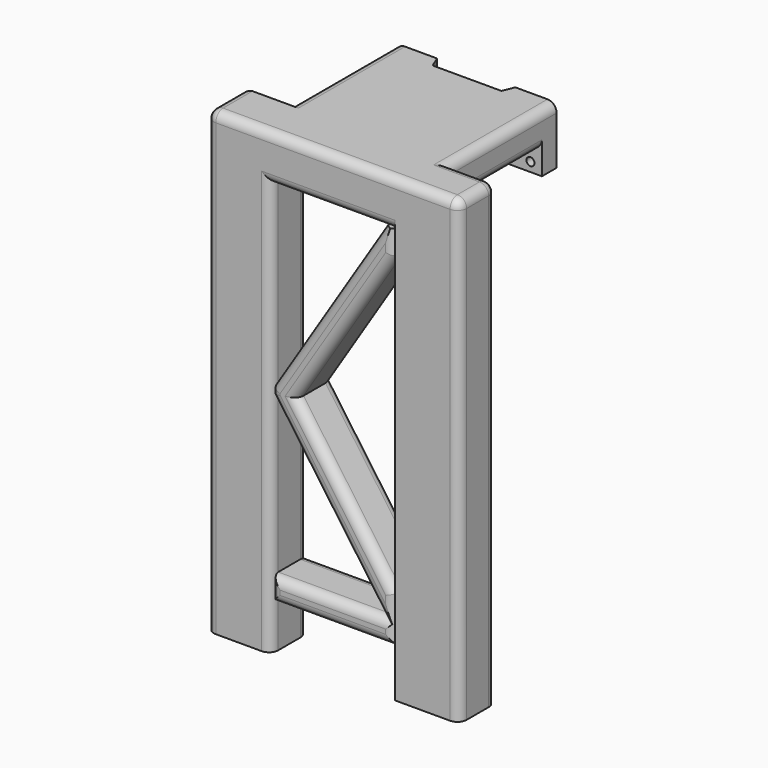
from build123d import *

# Parameters (mm, degrees)
F1_DEPTH         = 25
F2_R             = 1.75
F3_DEPTH         = 25
F4_W             = 70
F4_H             = 15
F5_DEPTH         = 50
F7_DEPTH         = 20
F7_DEPTH_BACK    = 90
F8_W             = 54
F8_H             = 180
F9_DEPTH         = 25
F12_DEPTH        = 20
F13_DEPTH        = 25
F14_T1_DEPTH     = 190
F14_T3_DEPTH     = 220
F14_T5_DEPTH     = 206
F14_T7_DEPTH     = 102
F14_T9_DEPTH     = 12
F14_T11_DEPTH    = 16
F14_T13_DEPTH    = 68
F14_T15_DEPTH    = 50
F14_T17_DEPTH    = 54
F14_T19_DEPTH    = 26
F14_S23_W        = 4
F14_S23_H        = 4
F14_T24_DEPTH    = 4
F14_S29_W        = 4
F14_S29_H        = 4
F14_T30_DEPTH    = 4
F14_S35_W        = 4
F14_S35_H        = 4
F14_T36_DEPTH    = 4
F14_T43_DEPTH    = 200
F14_T48_DEPTH    = 64
F14_T55_DEPTH    = 64
F14_T59_DEPTH    = 200
F14_T67_DEPTH    = 200
F14_T71_DEPTH    = 64
F14_T78_DEPTH    = 26
F14_T82_DEPTH    = 78
F14_2_T1_DEPTH   = 111.7221358849
F14_2_T3_DEPTH   = 30
F14_2_T5_DEPTH   = 74
F14_2_T7_DEPTH   = 40.2556151979
F14_2_T9_DEPTH   = 30.8068882586
F14_2_T11_DEPTH  = 23.071224869
F14_2_T16_DEPTH  = 100.4908539398
F14_2_T21_DEPTH  = 100.4908539398
F14_2_T26_DEPTH  = 94.5466591948
F14_2_T31_DEPTH  = 94.5466591948
F14_2_T36_DEPTH  = 104.9485186174
F14_2_T41_DEPTH  = 104.9485186174
F14_2_T46_DEPTH  = 69
F14_2_T51_DEPTH  = 69
F14_2_T57_DEPTH  = 94.5466591948
F14_2_T62_DEPTH  = 100.4908539398
F14_2_T70_DEPTH  = 100.4908539398
F14_2_T75_DEPTH  = 94.5466591948
F14_2_T83_DEPTH  = 59
F14_2_T88_DEPTH  = 104.9485186174
F14_2_T96_DEPTH  = 59
F14_2_T101_DEPTH = 104.9485186174


# Not quite as in the source:
# - a fillet or chamfer that OpenCascade refuses, or shapes differently, is made with other operations: its cross-section is extruded or revolved along the edge and cut away or added


with BuildPart() as f1:
    # F0 (on Top) → F1 (new body)
    with BuildSketch(Plane.XY):
        Polygon((-30.8332282406, 24.8506308587), (-48.8332282406, 24.8506308587), (-48.8332282406, 16.8506308587), (21.1667717594, 16.8506308587), (21.1667717594, 24.8506308587), (3.1667717594, 24.8506308587), (1.1667717594, 19.8506308587), (-28.8332282406, 19.8506308587), align=None)
    extrude(amount=F1_DEPTH)

    # F2 (on face) → F3 (cut)
    with BuildSketch(Plane(origin=(0, 24.8506308587, 0), x_dir=(-1, 0, 0), z_dir=(0, 1, 0))):
        with Locations((-16.1667717594, 4)):
            Circle(F2_R)
        with Locations((43.8332282406, 4)):
            Circle(F2_R)
    extrude(amount=-F3_DEPTH, mode=Mode.SUBTRACT)

    # F4 (on face) → F5 (join)
    with BuildSketch(Plane.XZ.offset(-16.8506308587)):
        with Locations((-13.8332282406, 17.5)):
            Rectangle(F4_W, F4_H)
    extrude(amount=F5_DEPTH)

    # F6 (on face) → F7 (join, two sides)
    with BuildSketch(Plane.YZ.offset(21.1667717594)) as f7_sk:
        Polygon((-33.1493691413, 10), (-33.1493691413, 25), (-53.1493691413, 25), (-53.1493691413, -175), (-33.1493691413, -175), align=None)
    extrude(amount=F7_DEPTH)
    extrude(f7_sk.sketch, amount=-F7_DEPTH_BACK)

    # F8 (on face) → F9 (cut)
    with BuildSketch(Plane(origin=(0, -33.1493691413, 0), x_dir=(-1, 0, 0), z_dir=(0, 1, 0))):
        with Locations((13.8332282406, -85)):
            Rectangle(F8_W, F8_H)
    extrude(amount=-F9_DEPTH, mode=Mode.SUBTRACT)

    # F10 (on face) → F13 (cut)
    with BuildSketch(Plane(origin=(0, 0, -175), x_dir=(1, 0, 0), z_dir=(0, 0, -1))):
        with BuildLine():
            Line((-62.8332282406, 37.1493691413), (-46.8332282406, 37.1493691413))
            ThreePointArc((-46.8332282406, 37.1493691413), (-45.4190146782, 37.7351555789), (-44.8332282406, 39.1493691413))
            Line((-44.8332282406, 39.1493691413), (-44.8332282406, 47.1493691413))
            ThreePointArc((-44.8332282406, 47.1493691413), (-45.4190146782, 48.5635827036), (-46.8332282406, 49.1493691413))
            Line((-46.8332282406, 49.1493691413), (-62.8332282406, 49.1493691413))
            ThreePointArc((-62.8332282406, 49.1493691413), (-64.247441803, 48.5635827036), (-64.8332282406, 47.1493691413))
            Line((-64.8332282406, 47.1493691413), (-64.8332282406, 39.1493691413))
            ThreePointArc((-64.8332282406, 39.1493691413), (-64.247441803, 37.7351555789), (-62.8332282406, 37.1493691413))
        make_face()
        with BuildLine():
            Line((19.1667717594, 37.1493691413), (35.1667717594, 37.1493691413))
            ThreePointArc((35.1667717594, 37.1493691413), (36.5809853218, 37.7351555789), (37.1667717594, 39.1493691413))
            Line((37.1667717594, 39.1493691413), (37.1667717594, 47.1493691413))
            ThreePointArc((37.1667717594, 47.1493691413), (36.5809853218, 48.5635827036), (35.1667717594, 49.1493691413))
            Line((35.1667717594, 49.1493691413), (19.1667717594, 49.1493691413))
            ThreePointArc((19.1667717594, 49.1493691413), (17.752558197, 48.5635827036), (17.1667717594, 47.1493691413))
            Line((17.1667717594, 47.1493691413), (17.1667717594, 39.1493691413))
            ThreePointArc((17.1667717594, 39.1493691413), (17.752558197, 37.7351555789), (19.1667717594, 37.1493691413))
        make_face()
    extrude(amount=-F13_DEPTH, mode=Mode.SUBTRACT)

    # F14: fillet of radius 4 on 17 edges, made by hand

    # F14_s2 → F14_t1 (cut)
    with BuildSketch(Plane.XY.offset(-185)):
        with BuildLine():
            ThreePointArc((13.1667717594, -37.1493691413), (14.3383446347, -34.3209420165), (17.1667717594, -33.1493691413))
            Line((17.1667717594, -33.1493691413), (13.1667717594, -33.1493691413))
            Line((13.1667717594, -33.1493691413), (13.1667717594, -37.1493691413))
        make_face()
        with BuildLine():
            ThreePointArc((-44.8332282406, -33.1493691413), (-42.0048011158, -34.3209420165), (-40.8332282406, -37.1493691413))
            Line((-40.8332282406, -37.1493691413), (-40.8332282406, -33.1493691413))
            Line((-40.8332282406, -33.1493691413), (-44.8332282406, -33.1493691413))
        make_face()
        with BuildLine():
            ThreePointArc((-44.8332282406, -53.1493691413), (-42.0048011158, -51.977796266), (-40.8332282406, -49.1493691413))
            Line((-40.8332282406, -49.1493691413), (-40.8332282406, -53.1493691413))
            Line((-40.8332282406, -53.1493691413), (-44.8332282406, -53.1493691413))
        make_face()
    extrude(amount=F14_T1_DEPTH, mode=Mode.SUBTRACT)

    # F14_s4 → F14_t3 (cut)
    with BuildSketch(Plane.XY.offset(-185)):
        with BuildLine():
            ThreePointArc((-64.8332282406, -33.1493691413), (-67.6616553653, -34.3209420165), (-68.8332282406, -37.1493691413))
            Line((-68.8332282406, -37.1493691413), (-68.8332282406, -33.1493691413))
            Line((-68.8332282406, -33.1493691413), (-64.8332282406, -33.1493691413))
        make_face()
    extrude(amount=F14_T3_DEPTH, mode=Mode.SUBTRACT)

    # F14_s6 → F14_t5 (cut)
    with BuildSketch(Plane.XY.offset(-185)):
        with BuildLine():
            ThreePointArc((41.1667717594, -37.1493691413), (39.9951988842, -34.3209420165), (37.1667717594, -33.1493691413))
            Line((37.1667717594, -33.1493691413), (41.1667717594, -33.1493691413))
            Line((41.1667717594, -33.1493691413), (41.1667717594, -37.1493691413))
        make_face()
        with BuildLine():
            ThreePointArc((37.1667717594, -53.1493691413), (39.9951988842, -51.977796266), (41.1667717594, -49.1493691413))
            Line((41.1667717594, -49.1493691413), (41.1667717594, -53.1493691413))
            Line((41.1667717594, -53.1493691413), (37.1667717594, -53.1493691413))
        make_face()
        with BuildLine():
            ThreePointArc((-64.8332282406, -53.1493691413), (-67.6616553653, -51.977796266), (-68.8332282406, -49.1493691413))
            Line((-68.8332282406, -49.1493691413), (-68.8332282406, -53.1493691413))
            Line((-68.8332282406, -53.1493691413), (-64.8332282406, -53.1493691413))
        make_face()
    extrude(amount=F14_T5_DEPTH, mode=Mode.SUBTRACT)

    # F14_s8 → F14_t7 (cut)
    with BuildSketch(Plane.YZ.offset(-64.8332282406)):
        with BuildLine():
            ThreePointArc((-53.1493691413, 21), (-51.977796266, 23.8284271247), (-49.1493691413, 25))
            Line((-49.1493691413, 25), (-53.1493691413, 25))
            Line((-53.1493691413, 25), (-53.1493691413, 21))
        make_face()
    extrude(amount=F14_T7_DEPTH, mode=Mode.SUBTRACT)

    # F14_s10 → F14_t9 (cut)
    with BuildSketch(Plane.XZ.offset(37.1493691413)):
        with BuildLine():
            ThreePointArc((41.1667717594, 21), (39.9951988842, 23.8284271247), (37.1667717594, 25))
            Line((37.1667717594, 25), (41.1667717594, 25))
            Line((41.1667717594, 25), (41.1667717594, 21))
        make_face()
    extrude(amount=F14_T9_DEPTH, mode=Mode.SUBTRACT)

    # F14_s12 → F14_t11 (cut)
    with BuildSketch(Plane.YZ.offset(21.1667717594)):
        with BuildLine():
            ThreePointArc((-33.1493691413, 21), (-34.3209420165, 23.8284271247), (-37.1493691413, 25))
            Line((-37.1493691413, 25), (-33.1493691413, 25))
            Line((-33.1493691413, 25), (-33.1493691413, 21))
        make_face()
    extrude(amount=F14_T11_DEPTH, mode=Mode.SUBTRACT)

    # F14_s14 → F14_t13 (cut)
    with BuildSketch(Plane.XZ.offset(-34.8506308587)):
        with BuildLine():
            ThreePointArc((17.1667717594, 25), (19.9951988842, 23.8284271247), (21.1667717594, 21))
            Line((21.1667717594, 21), (21.1667717594, 25))
            Line((21.1667717594, 25), (17.1667717594, 25))
        make_face()
        with BuildLine():
            ThreePointArc((-44.8332282406, 25), (-47.6616553653, 23.8284271247), (-48.8332282406, 21))
            Line((-48.8332282406, 21), (-48.8332282406, 25))
            Line((-48.8332282406, 25), (-44.8332282406, 25))
        make_face()
    extrude(amount=F14_T13_DEPTH, mode=Mode.SUBTRACT)

    # F14_s16 → F14_t15 (cut)
    with BuildSketch(Plane.XZ.offset(-16.8506308587)):
        with BuildLine():
            ThreePointArc((17.1667717594, 10), (19.9951988842, 11.1715728753), (21.1667717594, 14))
            Line((21.1667717594, 14), (21.1667717594, 10))
            Line((21.1667717594, 10), (17.1667717594, 10))
        make_face()
        with BuildLine():
            ThreePointArc((-48.8332282406, 14), (-47.6616553653, 11.1715728753), (-44.8332282406, 10))
            Line((-44.8332282406, 10), (-48.8332282406, 10))
            Line((-48.8332282406, 10), (-48.8332282406, 14))
        make_face()
    extrude(amount=F14_T15_DEPTH, mode=Mode.SUBTRACT)

    # F14_s18 → F14_t17 (cut)
    with BuildSketch(Plane.YZ.offset(-40.8332282406)):
        with BuildLine():
            ThreePointArc((-53.1493691413, 9), (-51.977796266, 6.1715728753), (-49.1493691413, 5))
            Line((-49.1493691413, 5), (-53.1493691413, 5))
            Line((-53.1493691413, 5), (-53.1493691413, 9))
        make_face()
        with BuildLine():
            ThreePointArc((-33.1493691413, 9), (-34.3209420165, 6.1715728753), (-37.1493691413, 5))
            Line((-37.1493691413, 5), (-33.1493691413, 5))
            Line((-33.1493691413, 5), (-33.1493691413, 9))
        make_face()
    extrude(amount=F14_T17_DEPTH, mode=Mode.SUBTRACT)

    # F14_s20 → F14_t19 (cut)
    with BuildSketch(Plane.XZ.offset(23.1493691413)):
        with BuildLine():
            ThreePointArc((-64.8332282406, 25), (-67.6616553653, 23.8284271247), (-68.8332282406, 21))
            Line((-68.8332282406, 21), (-68.8332282406, 25))
            Line((-68.8332282406, 25), (-64.8332282406, 25))
        make_face()
    extrude(amount=F14_T19_DEPTH, mode=Mode.SUBTRACT)


with BuildPart() as f12:
    # F11 (on face) → F12 (new body)
    with BuildSketch(Plane.XZ.offset(53.1493691413)):
        Polygon((-40.8332282406, -145), (-40.8332282406, -155), (13.1667717594, -155), (13.1667717594, -145), (13.1667717594, -134.7443848021), (-29.8332282406, -73.8493571142), (13.1667717594, -5.8068882586), (13.1667717594, 5), (8.1667717594, 5), (-40.8332282406, -72.5367668354), (-40.8332282406, -75.6079917045), (8.1667717594, -145), align=None)
    extrude(amount=-F12_DEPTH)

    # F14#2: fillet of radius 4 on 17 edges, made by hand

    # F14_2_s2 → F14_2_t1 (cut)
    with BuildSketch(Plane(origin=(9.9309720555, 0, 15.7146013207), x_dir=(0, 1, 0), z_dir=(-0.5342221867, 0, -0.8453441046))):
        with BuildLine():
            ThreePointArc((-33.1493691413, 8.2326214273), (-34.3209420165, 5.4041943026), (-37.1493691413, 4.2326214273))
            Line((-37.1493691413, 4.2326214273), (-33.1493691413, 4.2326214273))
            Line((-33.1493691413, 4.2326214273), (-33.1493691413, 8.2326214273))
        make_face()
        with BuildLine():
            ThreePointArc((-49.1493691413, 4.2326214273), (-51.977796266, 5.4041943026), (-53.1493691413, 8.2326214273))
            Line((-53.1493691413, 8.2326214273), (-53.1493691413, 4.2326214273))
            Line((-53.1493691413, 4.2326214273), (-49.1493691413, 4.2326214273))
        make_face()
    extrude(amount=F14_2_T1_DEPTH, mode=Mode.SUBTRACT)

    # F14_2_s4 → F14_2_t3 (cut)
    with BuildSketch(Plane.XY.offset(-165)):
        with BuildLine():
            ThreePointArc((-36.8332282406, -53.1493691413), (-39.6616553653, -51.977796266), (-40.8332282406, -49.1493691413))
            Line((-40.8332282406, -49.1493691413), (-40.8332282406, -53.1493691413))
            Line((-40.8332282406, -53.1493691413), (-36.8332282406, -53.1493691413))
        make_face()
    extrude(amount=F14_2_T3_DEPTH, mode=Mode.SUBTRACT)

    # F14_2_s6 → F14_2_t5 (cut)
    with BuildSketch(Plane.YZ.offset(-50.8332282406)):
        with BuildLine():
            ThreePointArc((-49.1493691413, -155), (-51.977796266, -153.8284271247), (-53.1493691413, -151))
            Line((-53.1493691413, -151), (-53.1493691413, -155))
            Line((-53.1493691413, -155), (-49.1493691413, -155))
        make_face()
        with BuildLine():
            ThreePointArc((-33.1493691413, -151), (-34.3209420165, -153.8284271247), (-37.1493691413, -155))
            Line((-37.1493691413, -155), (-33.1493691413, -155))
            Line((-33.1493691413, -155), (-33.1493691413, -151))
        make_face()
    extrude(amount=F14_2_T5_DEPTH, mode=Mode.SUBTRACT)

    # F14_2_s8 → F14_2_t7 (cut)
    with BuildSketch(Plane.XY.offset(-165)):
        with BuildLine():
            ThreePointArc((13.1667717594, -49.1493691413), (11.9951988842, -51.977796266), (9.1667717594, -53.1493691413))
            Line((9.1667717594, -53.1493691413), (13.1667717594, -53.1493691413))
            Line((13.1667717594, -53.1493691413), (13.1667717594, -49.1493691413))
        make_face()
    extrude(amount=F14_2_T7_DEPTH, mode=Mode.SUBTRACT)

    # F14_2_s10 → F14_2_t9 (cut)
    with BuildSketch(Plane.XY.offset(-15.8068882586)):
        with BuildLine():
            ThreePointArc((13.1667717594, -49.1493691413), (11.9951988842, -51.977796266), (9.1667717594, -53.1493691413))
            Line((9.1667717594, -53.1493691413), (13.1667717594, -53.1493691413))
            Line((13.1667717594, -53.1493691413), (13.1667717594, -49.1493691413))
        make_face()
    extrude(amount=F14_2_T9_DEPTH, mode=Mode.SUBTRACT)

    # F14_2_s12 → F14_2_t11 (cut)
    with BuildSketch(Plane.XY.offset(-85.6079917045)):
        with BuildLine():
            ThreePointArc((-40.8332282406, -49.1493691413), (-39.6616553653, -51.977796266), (-36.8332282406, -53.1493691413))
            Line((-36.8332282406, -53.1493691413), (-40.8332282406, -53.1493691413))
            Line((-40.8332282406, -53.1493691413), (-40.8332282406, -49.1493691413))
        make_face()
    extrude(amount=F14_2_T11_DEPTH, mode=Mode.SUBTRACT)


with BuildPart() as f14_tool22:
    # F14_s23 → F14_t24 (new body)
    with BuildSketch(Plane.YZ.offset(37.1667717594)):
        with Locations((-35.1493691413, 23)):
            Rectangle(F14_S23_W, F14_S23_H)
    extrude(amount=F14_T24_DEPTH)

    # F14_s25 → F14_t26 (revolve, cut)
    with BuildSketch(Plane(origin=(37.1667717594, -37.1493691413, 21), x_dir=(0, -0.7071067812, -0.7071067812), z_dir=(0, -0.7071067812, 0.7071067812))):
        with BuildLine():
            ThreePointArc((0, -4), (4, 0), (0, 4))
            Line((0, 4), (0, -4))
        make_face()
    revolve(axis=Axis((37.1667717594, -37.1493691413, 21), (1, 0, 0)), mode=Mode.SUBTRACT)


with BuildPart() as f1_1:
    add(f1.part)

    # F14_t21: cut F14_tool22
    add(f14_tool22.part, mode=Mode.SUBTRACT)


with BuildPart() as f14_tool28:
    # F14_s29 → F14_t30 (new body)
    with BuildSketch(Plane.XZ.offset(49.1493691413)):
        with Locations((39.1667717594, 23)):
            Rectangle(F14_S29_W, F14_S29_H)
    extrude(amount=F14_T30_DEPTH)

    # F14_s31 → F14_t32 (revolve, cut)
    with BuildSketch(Plane(origin=(37.1667717594, -49.1493691413, 21), x_dir=(-0.7071067812, 0, -0.7071067812), z_dir=(-0.7071067812, 0, 0.7071067812))):
        with BuildLine():
            ThreePointArc((0, -4), (4, 0), (0, 4))
            Line((0, 4), (0, -4))
        make_face()
    revolve(axis=Axis((37.1667717594, -49.1493691413, 21), (0, -1, 0)), mode=Mode.SUBTRACT)


with BuildPart() as f1_2:
    add(f1_1.part)

    # F14_t27: cut F14_tool28
    add(f14_tool28.part, mode=Mode.SUBTRACT)


with BuildPart() as f14_tool34:
    # F14_s35 → F14_t36 (new body)
    with BuildSketch(Plane.XZ.offset(49.1493691413)):
        with Locations((-66.8332282406, 23)):
            Rectangle(F14_S35_W, F14_S35_H)
    extrude(amount=F14_T36_DEPTH)

    # F14_s37 → F14_t38 (revolve, cut)
    with BuildSketch(Plane(origin=(-64.8332282406, -49.1493691413, 21), x_dir=(0.7071067812, 0, -0.7071067812), z_dir=(-0.7071067812, 0, -0.7071067812))):
        with BuildLine():
            ThreePointArc((0, -4), (4, 0), (0, 4))
            Line((0, 4), (0, -4))
        make_face()
    revolve(axis=Axis((-64.8332282406, -49.1493691413, 21), (0, -1, 0)), mode=Mode.SUBTRACT)


with BuildPart() as f1_3:
    add(f1_2.part)

    # F14_t33: cut F14_tool34
    add(f14_tool34.part, mode=Mode.SUBTRACT)


with BuildPart() as f14_tool41:
    # F14_s42 → F14_t43 (new body)
    with BuildSketch(Plane.XY.offset(15)):
        with BuildLine():
            ThreePointArc((13.1667717594, -37.1493691413), (14.3383446347, -34.3209420165), (17.1667717594, -33.1493691413))
            Line((17.1667717594, -33.1493691413), (13.1667717594, -33.1493691413))
            Line((13.1667717594, -33.1493691413), (13.1667717594, -37.1493691413))
        make_face()
    extrude(amount=-F14_T43_DEPTH)

    split(bisect_by=Plane.XY.offset(5), keep=Keep.TOP)

    split(bisect_by=Plane.XY.offset(10), keep=Keep.BOTTOM)


with BuildPart() as f14_tool46:
    # F14_s47 → F14_t48 (new body)
    with BuildSketch(Plane.YZ.offset(-40.8332282406)):
        with BuildLine():
            ThreePointArc((-33.1493691413, 9), (-34.3209420165, 6.1715728753), (-37.1493691413, 5))
            Line((-37.1493691413, 5), (-33.1493691413, 5))
            Line((-33.1493691413, 5), (-33.1493691413, 9))
        make_face()
    extrude(amount=F14_T48_DEPTH)

    split(bisect_by=Plane.YZ.offset(13.1667717594), keep=Keep.TOP)


with BuildPart() as f14_tool41_1:
    add(f14_tool41.part)

    # F14_t50: intersect F14_tool46
    add(f14_tool46.part, mode=Mode.INTERSECT)


with BuildPart() as f1_4:
    add(f1_3.part)

    # F14_t39: cut F14_tool41
    add(f14_tool41_1.part, mode=Mode.SUBTRACT)


with BuildPart() as f14_tool53:
    # F14_s54 → F14_t55 (new body)
    with BuildSketch(Plane.YZ.offset(-50.8332282406)):
        with BuildLine():
            ThreePointArc((-33.1493691413, 9), (-34.3209420165, 6.1715728753), (-37.1493691413, 5))
            Line((-37.1493691413, 5), (-33.1493691413, 5))
            Line((-33.1493691413, 5), (-33.1493691413, 9))
        make_face()
    extrude(amount=F14_T55_DEPTH)

    split(bisect_by=Plane.YZ.offset(-40.8332282406), keep=Keep.BOTTOM)


with BuildPart() as f14_tool57:
    # F14_s58 → F14_t59 (new body)
    with BuildSketch(Plane.XY.offset(-185)):
        with BuildLine():
            ThreePointArc((-44.8332282406, -33.1493691413), (-42.0048011158, -34.3209420165), (-40.8332282406, -37.1493691413))
            Line((-40.8332282406, -37.1493691413), (-40.8332282406, -33.1493691413))
            Line((-40.8332282406, -33.1493691413), (-44.8332282406, -33.1493691413))
        make_face()
    extrude(amount=F14_T59_DEPTH)

    split(bisect_by=Plane.XY.offset(10), keep=Keep.BOTTOM)

    split(bisect_by=Plane.XY.offset(5), keep=Keep.TOP)


with BuildPart() as f14_tool53_1:
    add(f14_tool53.part)

    # F14_t62: intersect F14_tool57
    add(f14_tool57.part, mode=Mode.INTERSECT)


with BuildPart() as f1_5:
    add(f1_4.part)

    # F14_t51: cut F14_tool53
    add(f14_tool53_1.part, mode=Mode.SUBTRACT)


with BuildPart() as f14_tool65:
    # F14_s66 → F14_t67 (new body)
    with BuildSketch(Plane.XY.offset(-185)):
        with BuildLine():
            ThreePointArc((-44.8332282406, -53.1493691413), (-42.0048011158, -51.977796266), (-40.8332282406, -49.1493691413))
            Line((-40.8332282406, -49.1493691413), (-40.8332282406, -53.1493691413))
            Line((-40.8332282406, -53.1493691413), (-44.8332282406, -53.1493691413))
        make_face()
    extrude(amount=F14_T67_DEPTH)

    split(bisect_by=Plane.XY.offset(5), keep=Keep.TOP)


with BuildPart() as f14_tool69:
    # F14_s70 → F14_t71 (new body)
    with BuildSketch(Plane.YZ.offset(-50.8332282406)):
        with BuildLine():
            ThreePointArc((-53.1493691413, 9), (-51.977796266, 6.1715728753), (-49.1493691413, 5))
            Line((-49.1493691413, 5), (-53.1493691413, 5))
            Line((-53.1493691413, 5), (-53.1493691413, 9))
        make_face()
    extrude(amount=F14_T71_DEPTH)

    split(bisect_by=Plane.YZ.offset(-40.8332282406), keep=Keep.BOTTOM)


with BuildPart() as f14_tool65_1:
    add(f14_tool65.part)

    # F14_t73: intersect F14_tool69
    add(f14_tool69.part, mode=Mode.INTERSECT)


with BuildPart() as f1_6:
    add(f1_5.part)

    # F14_t63: cut F14_tool65
    add(f14_tool65_1.part, mode=Mode.SUBTRACT)


with BuildPart() as f14_tool76:
    # F14_s77 → F14_t78 (new body)
    with BuildSketch(Plane.YZ.offset(11.1667717594)):
        with BuildLine():
            ThreePointArc((-33.1493691413, 21), (-34.3209420165, 23.8284271247), (-37.1493691413, 25))
            Line((-37.1493691413, 25), (-33.1493691413, 25))
            Line((-33.1493691413, 25), (-33.1493691413, 21))
        make_face()
    extrude(amount=F14_T78_DEPTH)

    split(bisect_by=Plane.YZ.offset(21.1667717594), keep=Keep.BOTTOM)


with BuildPart() as f14_tool80:
    # F14_s81 → F14_t82 (new body)
    with BuildSketch(Plane.XZ.offset(-34.8506308587)):
        with BuildLine():
            ThreePointArc((17.1667717594, 25), (19.9951988842, 23.8284271247), (21.1667717594, 21))
            Line((21.1667717594, 21), (21.1667717594, 25))
            Line((21.1667717594, 25), (17.1667717594, 25))
        make_face()
    extrude(amount=F14_T82_DEPTH)

    split(bisect_by=Plane.XZ.offset(33.1493691413), keep=Keep.TOP)


with BuildPart() as f14_tool76_1:
    add(f14_tool76.part)

    # F14_t84: intersect F14_tool80
    add(f14_tool80.part, mode=Mode.INTERSECT)


with BuildPart() as f1_7:
    add(f1_6.part)

    # F14_t74: cut F14_tool76
    add(f14_tool76_1.part, mode=Mode.SUBTRACT)


with BuildPart() as f14_2_tool14:
    # F14_2_s15 → F14_2_t16 (new body)
    with BuildSketch(Plane(origin=(-47.2069127246, 0, -74.6994160194), x_dir=(0, 1, 0), z_dir=(0.5342221867, 0, 0.8453441046))):
        with BuildLine():
            ThreePointArc((-33.1493691413, -10.2326214273), (-34.3209420165, -13.0610485521), (-37.1493691413, -14.2326214273))
            Line((-37.1493691413, -14.2326214273), (-33.1493691413, -14.2326214273))
            Line((-33.1493691413, -14.2326214273), (-33.1493691413, -10.2326214273))
        make_face()
    extrude(amount=F14_2_T16_DEPTH)

    split(bisect_by=Plane(origin=(-54.7039857102, 0, -38.6282997948), x_dir=(0, 1, 0), z_dir=(0.8168713172, 0, 0.5768199469)), keep=Keep.TOP)


with BuildPart() as f12_1:
    add(f12.part)

    # F14_2_t13: cut F14_2_tool14
    add(f14_2_tool14.part, mode=Mode.SUBTRACT)


with BuildPart() as f14_2_tool19:
    # F14_2_s20 → F14_2_t21 (new body)
    with BuildSketch(Plane(origin=(-47.2069127246, 0, -74.6994160194), x_dir=(0, 1, 0), z_dir=(0.5342221867, 0, 0.8453441046))):
        with BuildLine():
            ThreePointArc((-49.1493691413, -14.2326214273), (-51.977796266, -13.0610485521), (-53.1493691413, -10.2326214273))
            Line((-53.1493691413, -10.2326214273), (-53.1493691413, -14.2326214273))
            Line((-53.1493691413, -14.2326214273), (-49.1493691413, -14.2326214273))
        make_face()
    extrude(amount=F14_2_T21_DEPTH)

    split(bisect_by=Plane(origin=(-54.7039857102, 0, -38.6282997948), x_dir=(0, 1, 0), z_dir=(0.8168713172, 0, 0.5768199469)), keep=Keep.TOP)


with BuildPart() as f12_2:
    add(f12_1.part)

    # F14_2_t18: cut F14_2_tool19
    add(f14_2_tool19.part, mode=Mode.SUBTRACT)


with BuildPart() as f14_2_tool24:
    # F14_2_s25 → F14_2_t26 (new body)
    with BuildSketch(Plane(origin=(73.6389569389, 0, -104.2847981791), x_dir=(0, 1, 0), z_dir=(-0.5768199469, 0, 0.8168713172))):
        with BuildLine():
            ThreePointArc((-33.1493691413, 70.9676906995), (-34.3209420165, 68.1392635747), (-37.1493691413, 66.9676906995))
            Line((-37.1493691413, 66.9676906995), (-33.1493691413, 66.9676906995))
            Line((-33.1493691413, 66.9676906995), (-33.1493691413, 70.9676906995))
        make_face()
    extrude(amount=F14_2_T26_DEPTH)

    split(bisect_by=Plane(origin=(12.0314626172, 0, -7.6033821412), x_dir=(0, 1, 0), z_dir=(0.8453441046, 0, -0.5342221867)), keep=Keep.TOP)


with BuildPart() as f12_3:
    add(f12_2.part)

    # F14_2_t23: cut F14_2_tool24
    add(f14_2_tool24.part, mode=Mode.SUBTRACT)


with BuildPart() as f14_2_tool29:
    # F14_2_s30 → F14_2_t31 (new body)
    with BuildSketch(Plane(origin=(73.6389569389, 0, -104.2847981791), x_dir=(0, 1, 0), z_dir=(-0.5768199469, 0, 0.8168713172))):
        with BuildLine():
            ThreePointArc((-49.1493691413, 66.9676906995), (-51.977796266, 68.1392635747), (-53.1493691413, 70.9676906995))
            Line((-53.1493691413, 70.9676906995), (-53.1493691413, 66.9676906995))
            Line((-53.1493691413, 66.9676906995), (-49.1493691413, 66.9676906995))
        make_face()
    extrude(amount=F14_2_T31_DEPTH)

    split(bisect_by=Plane(origin=(12.0314626172, 0, -7.6033821412), x_dir=(0, 1, 0), z_dir=(0.8453441046, 0, -0.5342221867)), keep=Keep.TOP)


with BuildPart() as f12_4:
    add(f12_3.part)

    # F14_2_t28: cut F14_2_tool29
    add(f14_2_tool29.part, mode=Mode.SUBTRACT)


with BuildPart() as f14_2_tool34:
    # F14_2_s35 → F14_2_t36 (new body)
    with BuildSketch(Plane(origin=(16.2712711723, 0, -23.0427792687), x_dir=(0, 1, 0), z_dir=(0.5768199469, 0, -0.8168713172))):
        with BuildLine():
            ThreePointArc((-33.1493691413, -72.9676906995), (-34.3209420165, -75.7961178242), (-37.1493691413, -76.9676906995))
            Line((-37.1493691413, -76.9676906995), (-33.1493691413, -76.9676906995))
            Line((-33.1493691413, -76.9676906995), (-33.1493691413, -72.9676906995))
        make_face()
    extrude(amount=F14_2_T36_DEPTH)

    split(bisect_by=Plane.XY.offset(-145), keep=Keep.TOP)


with BuildPart() as f12_5:
    add(f12_4.part)

    # F14_2_t33: cut F14_2_tool34
    add(f14_2_tool34.part, mode=Mode.SUBTRACT)


with BuildPart() as f14_2_tool39:
    # F14_2_s40 → F14_2_t41 (new body)
    with BuildSketch(Plane(origin=(16.2712711723, 0, -23.0427792687), x_dir=(0, 1, 0), z_dir=(0.5768199469, 0, -0.8168713172))):
        with BuildLine():
            ThreePointArc((-53.1493691413, -72.9676906995), (-51.977796266, -75.7961178242), (-49.1493691413, -76.9676906995))
            Line((-49.1493691413, -76.9676906995), (-53.1493691413, -76.9676906995))
            Line((-53.1493691413, -76.9676906995), (-53.1493691413, -72.9676906995))
        make_face()
    extrude(amount=F14_2_T41_DEPTH)

    split(bisect_by=Plane.XY.offset(-145), keep=Keep.TOP)


with BuildPart() as f12_6:
    add(f12_5.part)

    # F14_2_t38: cut F14_2_tool39
    add(f14_2_tool39.part, mode=Mode.SUBTRACT)


with BuildPart() as f14_2_tool44:
    # F14_2_s45 → F14_2_t46 (new body)
    with BuildSketch(Plane.YZ.offset(18.1667717594)):
        with BuildLine():
            ThreePointArc((-49.1493691413, -145), (-51.977796266, -146.1715728753), (-53.1493691413, -149))
            Line((-53.1493691413, -149), (-53.1493691413, -145))
            Line((-53.1493691413, -145), (-49.1493691413, -145))
        make_face()
    extrude(amount=-F14_2_T46_DEPTH)

    split(bisect_by=Plane(origin=(-62.8726988821, 0, -44.396499264), x_dir=(0, 1, 0), z_dir=(-0.8168713172, 0, -0.5768199469)), keep=Keep.TOP)


with BuildPart() as f12_7:
    add(f12_6.part)

    # F14_2_t43: cut F14_2_tool44
    add(f14_2_tool44.part, mode=Mode.SUBTRACT)


with BuildPart() as f14_2_tool49:
    # F14_2_s50 → F14_2_t51 (new body)
    with BuildSketch(Plane.YZ.offset(18.1667717594)):
        with BuildLine():
            ThreePointArc((-37.1493691413, -145), (-34.3209420165, -146.1715728753), (-33.1493691413, -149))
            Line((-33.1493691413, -149), (-33.1493691413, -145))
            Line((-33.1493691413, -145), (-37.1493691413, -145))
        make_face()
    extrude(amount=-F14_2_T51_DEPTH)

    split(bisect_by=Plane(origin=(-62.8726988821, 0, -44.396499264), x_dir=(0, 1, 0), z_dir=(-0.8168713172, 0, -0.5768199469)), keep=Keep.TOP)


with BuildPart() as f12_8:
    add(f12_7.part)

    # F14_2_t48: cut F14_2_tool49
    add(f14_2_tool49.part, mode=Mode.SUBTRACT)


with BuildPart() as f14_2_tool55:
    # F14_2_s56 → F14_2_t57 (new body)
    with BuildSketch(Plane(origin=(73.6389569389, 0, -104.2847981791), x_dir=(0, 1, 0), z_dir=(-0.5768199469, 0, 0.8168713172))):
        with BuildLine():
            ThreePointArc((-33.1493691413, 70.9676906995), (-34.3209420165, 68.1392635747), (-37.1493691413, 66.9676906995))
            Line((-37.1493691413, 66.9676906995), (-33.1493691413, 66.9676906995))
            Line((-33.1493691413, 66.9676906995), (-33.1493691413, 70.9676906995))
        make_face()
    extrude(amount=F14_2_T57_DEPTH)

    split(bisect_by=Plane(origin=(3.5780215708, 0, -2.2611602743), x_dir=(0, 1, 0), z_dir=(0.8453441046, 0, -0.5342221867)), keep=Keep.TOP)

    split(bisect_by=Plane(origin=(12.0314626172, 0, -7.6033821412), x_dir=(0, 1, 0), z_dir=(-0.8453441046, 0, 0.5342221867)), keep=Keep.TOP)


with BuildPart() as f14_2_tool60:
    # F14_2_s61 → F14_2_t62 (new body)
    with BuildSketch(Plane(origin=(-47.2069127246, 0, -74.6994160194), x_dir=(0, 1, 0), z_dir=(0.5342221867, 0, 0.8453441046))):
        with BuildLine():
            ThreePointArc((-33.1493691413, -10.2326214273), (-34.3209420165, -13.0610485521), (-37.1493691413, -14.2326214273))
            Line((-37.1493691413, -14.2326214273), (-33.1493691413, -14.2326214273))
            Line((-33.1493691413, -14.2326214273), (-33.1493691413, -10.2326214273))
        make_face()
    extrude(amount=F14_2_T62_DEPTH)

    split(bisect_by=Plane(origin=(-54.7039857102, 0, -38.6282997948), x_dir=(0, 1, 0), z_dir=(-0.8168713172, 0, -0.5768199469)), keep=Keep.TOP)

    split(bisect_by=Plane(origin=(-62.8726988821, 0, -44.396499264), x_dir=(0, 1, 0), z_dir=(0.8168713172, 0, 0.5768199469)), keep=Keep.TOP)


with BuildPart() as f14_2_tool55_1:
    add(f14_2_tool55.part)

    # F14_2_t65: intersect F14_2_tool60
    add(f14_2_tool60.part, mode=Mode.INTERSECT)


with BuildPart() as f12_9:
    add(f12_8.part)

    # F14_2_t53: cut F14_2_tool55
    add(f14_2_tool55_1.part, mode=Mode.SUBTRACT)


with BuildPart() as f14_2_tool68:
    # F14_2_s69 → F14_2_t70 (new body)
    with BuildSketch(Plane(origin=(-47.2069127246, 0, -74.6994160194), x_dir=(0, 1, 0), z_dir=(0.5342221867, 0, 0.8453441046))):
        with BuildLine():
            ThreePointArc((-49.1493691413, -14.2326214273), (-51.977796266, -13.0610485521), (-53.1493691413, -10.2326214273))
            Line((-53.1493691413, -10.2326214273), (-53.1493691413, -14.2326214273))
            Line((-53.1493691413, -14.2326214273), (-49.1493691413, -14.2326214273))
        make_face()
    extrude(amount=F14_2_T70_DEPTH)

    split(bisect_by=Plane(origin=(-54.7039857102, 0, -38.6282997948), x_dir=(0, 1, 0), z_dir=(-0.8168713172, 0, -0.5768199469)), keep=Keep.TOP)

    split(bisect_by=Plane(origin=(-62.8726988821, 0, -44.396499264), x_dir=(0, 1, 0), z_dir=(0.8168713172, 0, 0.5768199469)), keep=Keep.TOP)


with BuildPart() as f14_2_tool73:
    # F14_2_s74 → F14_2_t75 (new body)
    with BuildSketch(Plane(origin=(73.6389569389, 0, -104.2847981791), x_dir=(0, 1, 0), z_dir=(-0.5768199469, 0, 0.8168713172))):
        with BuildLine():
            ThreePointArc((-49.1493691413, 66.9676906995), (-51.977796266, 68.1392635747), (-53.1493691413, 70.9676906995))
            Line((-53.1493691413, 70.9676906995), (-53.1493691413, 66.9676906995))
            Line((-53.1493691413, 66.9676906995), (-49.1493691413, 66.9676906995))
        make_face()
    extrude(amount=F14_2_T75_DEPTH)

    split(bisect_by=Plane(origin=(3.5780215708, 0, -2.2611602743), x_dir=(0, 1, 0), z_dir=(0.8453441046, 0, -0.5342221867)), keep=Keep.TOP)

    split(bisect_by=Plane(origin=(12.0314626172, 0, -7.6033821412), x_dir=(0, 1, 0), z_dir=(-0.8453441046, 0, 0.5342221867)), keep=Keep.TOP)


with BuildPart() as f14_2_tool68_1:
    add(f14_2_tool68.part)

    # F14_2_t78: intersect F14_2_tool73
    add(f14_2_tool73.part, mode=Mode.INTERSECT)


with BuildPart() as f12_10:
    add(f12_9.part)

    # F14_2_t66: cut F14_2_tool68
    add(f14_2_tool68_1.part, mode=Mode.SUBTRACT)


with BuildPart() as f14_2_tool81:
    # F14_2_s82 → F14_2_t83 (new body)
    with BuildSketch(Plane.YZ.offset(18.1667717594)):
        with BuildLine():
            ThreePointArc((-37.1493691413, -145), (-34.3209420165, -146.1715728753), (-33.1493691413, -149))
            Line((-33.1493691413, -149), (-33.1493691413, -145))
            Line((-33.1493691413, -145), (-37.1493691413, -145))
        make_face()
    extrude(amount=-F14_2_T83_DEPTH)

    split(bisect_by=Plane.YZ.offset(13.1667717594), keep=Keep.BOTTOM)

    split(bisect_by=Plane(origin=(-62.8726988821, 0, -44.396499264), x_dir=(0, 1, 0), z_dir=(0.8168713172, 0, 0.5768199469)), keep=Keep.TOP)


with BuildPart() as f14_2_tool86:
    # F14_2_s87 → F14_2_t88 (new body)
    with BuildSketch(Plane(origin=(16.2712711723, 0, -23.0427792687), x_dir=(0, 1, 0), z_dir=(0.5768199469, 0, -0.8168713172))):
        with BuildLine():
            ThreePointArc((-33.1493691413, -72.9676906995), (-34.3209420165, -75.7961178242), (-37.1493691413, -76.9676906995))
            Line((-37.1493691413, -76.9676906995), (-33.1493691413, -76.9676906995))
            Line((-33.1493691413, -76.9676906995), (-33.1493691413, -72.9676906995))
        make_face()
    extrude(amount=F14_2_T88_DEPTH)

    split(bisect_by=Plane.XY.offset(-145), keep=Keep.BOTTOM)

    split(bisect_by=Plane.YZ.offset(13.1667717594), keep=Keep.BOTTOM)


with BuildPart() as f14_2_tool81_1:
    add(f14_2_tool81.part)

    # F14_2_t91: intersect F14_2_tool86
    add(f14_2_tool86.part, mode=Mode.INTERSECT)


with BuildPart() as f12_11:
    add(f12_10.part)

    # F14_2_t79: cut F14_2_tool81
    add(f14_2_tool81_1.part, mode=Mode.SUBTRACT)


with BuildPart() as f14_2_tool94:
    # F14_2_s95 → F14_2_t96 (new body)
    with BuildSketch(Plane.YZ.offset(18.1667717594)):
        with BuildLine():
            ThreePointArc((-49.1493691413, -145), (-51.977796266, -146.1715728753), (-53.1493691413, -149))
            Line((-53.1493691413, -149), (-53.1493691413, -145))
            Line((-53.1493691413, -145), (-49.1493691413, -145))
        make_face()
    extrude(amount=-F14_2_T96_DEPTH)

    split(bisect_by=Plane.YZ.offset(13.1667717594), keep=Keep.BOTTOM)

    split(bisect_by=Plane(origin=(-62.8726988821, 0, -44.396499264), x_dir=(0, 1, 0), z_dir=(0.8168713172, 0, 0.5768199469)), keep=Keep.TOP)


with BuildPart() as f14_2_tool99:
    # F14_2_s100 → F14_2_t101 (new body)
    with BuildSketch(Plane(origin=(16.2712711723, 0, -23.0427792687), x_dir=(0, 1, 0), z_dir=(0.5768199469, 0, -0.8168713172))):
        with BuildLine():
            ThreePointArc((-53.1493691413, -72.9676906995), (-51.977796266, -75.7961178242), (-49.1493691413, -76.9676906995))
            Line((-49.1493691413, -76.9676906995), (-53.1493691413, -76.9676906995))
            Line((-53.1493691413, -76.9676906995), (-53.1493691413, -72.9676906995))
        make_face()
    extrude(amount=F14_2_T101_DEPTH)

    split(bisect_by=Plane.XY.offset(-145), keep=Keep.BOTTOM)

    split(bisect_by=Plane.YZ.offset(13.1667717594), keep=Keep.BOTTOM)


with BuildPart() as f14_2_tool94_1:
    add(f14_2_tool94.part)

    # F14_2_t104: intersect F14_2_tool99
    add(f14_2_tool99.part, mode=Mode.INTERSECT)


with BuildPart() as f12_12:
    add(f12_11.part)

    # F14_2_t92: cut F14_2_tool94
    add(f14_2_tool94_1.part, mode=Mode.SUBTRACT)


solid = Compound([f1_7.part, f12_12.part])
